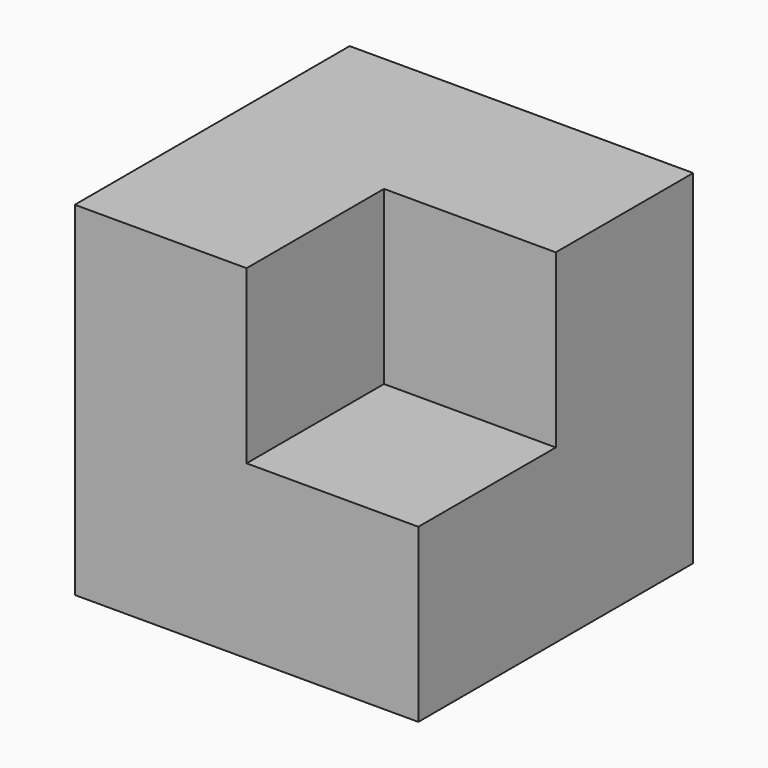
from build123d import *

# Parameters (mm, degrees)
F0_W     = 50.8
F0_H     = 50.8
F1_DEPTH = 50.8
F2_W     = 25.4
F2_H     = 25.4
F3_DEPTH = 25.4


# Not quite as in the source:
# - a feature names something its author has since deleted; it is built from what else it names


with BuildPart() as f1:
    # F0 (on Front) → F1 (new body)
    with BuildSketch(Plane.XZ):
        with Locations((-25.4, 25.4)):
            Rectangle(F0_W, F0_H)
    extrude(amount=F1_DEPTH)

    # F2 (on face) → F3 (cut)
    with BuildSketch(Plane.XY.offset(50.8)):
        with Locations((-12.7, -38.1)):
            Rectangle(F2_W, F2_H)
    extrude(amount=-F3_DEPTH, mode=Mode.SUBTRACT)


solid = f1.part
